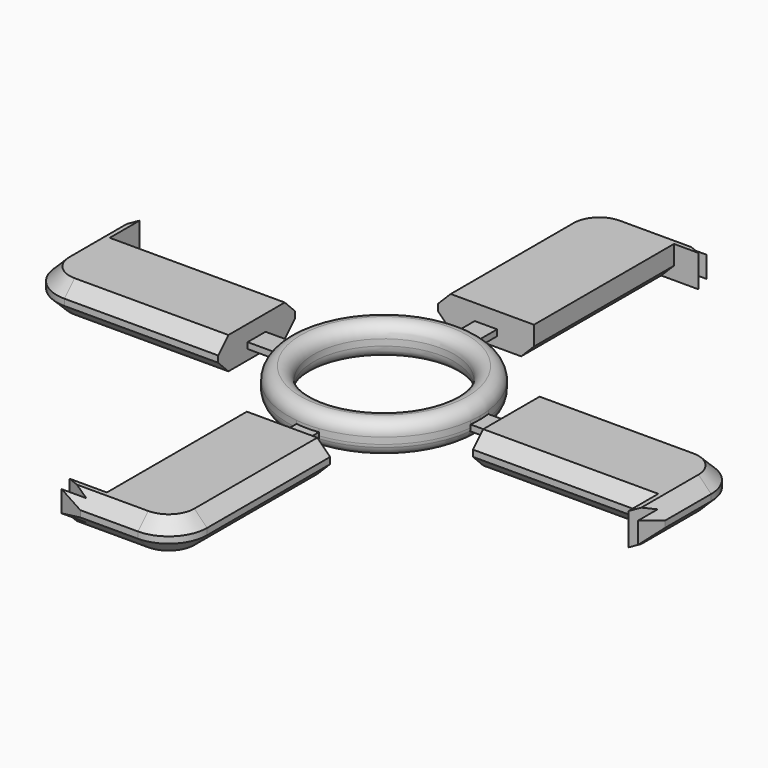
from build123d import *
from build123d import SkipClean  # not in build123d's __all__

# Parameters (mm, degrees)
F1_DEPTH     = 12.7
F0_R         = 27.94
F2_DEPTH     = 6.35
F3_DEPTH     = 3.937
F4_R         = 15.24
F5_SIZE      = 5.08
F6_T9_ANGLE  = 13.3995303555
F6_T16_ANGLE = 76.6004696445
F6_T21_ANGLE = 76.6004696445
F6_T25_ANGLE = 76.6004696445
F6_T30_ANGLE = 76.6004696445
F6_T34_ANGLE = 76.6004696445
F6_T39_ANGLE = 76.6004696445
F6_T43_ANGLE = 76.6004696445
F6_T48_ANGLE = 76.6004696445
F6_T52_ANGLE = 13.3995303555
F6_T56_ANGLE = 13.3995303555
F6_T60_ANGLE = 13.3995303555


# Not quite as in the source:
# - a fillet or chamfer that OpenCascade refuses, or shapes differently, is made with other operations: its cross-section is extruded or revolved along the edge and cut away or added


with BuildPart() as f1:
    # F0 (on Top) → F1 (new body)
    with BuildSketch(Plane.XY):
        Polygon((-50.5398199652, -4.445), (-50.5398199652, 4.445), (-50.5398199652, 19.05), (-119.9662685394, 19.05), (-123.7786710262, 19.05), (-126.7398199652, 19.05), (-126.7398199652, -19.05), (-50.5398199652, -19.05), align=None)
        Polygon((-126.7398199652, 19.05), (-123.7786710262, 19.05), (-123.7786710262, 28.8333185017), align=None)
        Polygon((-123.7786710262, 19.05), (-119.9662685394, 19.05), (-119.9662685394, 28.8333185017), align=None)
    extrude(amount=F1_DEPTH)



with BuildPart() as f1b:
    # F0 (on Top) → F1, piece 2 (new body)
    with BuildSketch(Plane.XY):
        with BuildLine():
            ThreePointArc((37.8398199652, -4.445), (38.0348993733, -2.2263040364), (38.1, 0))
            ThreePointArc((38.1, 0), (38.0348993733, 2.2263040364), (37.8398199652, 4.445))
            ThreePointArc((37.8398199652, 4.445), (26.9407683632, 26.9407683632), (4.445, 37.8398199652))
            ThreePointArc((4.445, 37.8398199652), (0, 38.1), (-4.445, 37.8398199652))
            ThreePointArc((-4.445, 37.8398199652), (-26.9407683632, 26.9407683632), (-37.8398199652, 4.445))
            ThreePointArc((-37.8398199652, 4.445), (-38.1, 0), (-37.8398199652, -4.445))
            ThreePointArc((-37.8398199652, -4.445), (-26.9407683632, -26.9407683632), (-4.445, -37.8398199652))
            ThreePointArc((-4.445, -37.8398199652), (0, -38.1), (4.445, -37.8398199652))
            ThreePointArc((4.445, -37.8398199652), (26.9407683632, -26.9407683632), (37.8398199652, -4.445))
        make_face()
        Circle(F0_R, mode=Mode.SUBTRACT)
    extrude(amount=F1_DEPTH)


with BuildPart() as f1c:
    # F0 (on Top) → F1, piece 3 (new body)
    with BuildSketch(Plane.XY):
        Polygon((50.5398199652, 19.05), (50.5398199652, 4.445), (50.5398199652, -4.445), (50.5398199652, -19.05), (119.9662685394, -19.05), (123.7786710262, -19.05), (126.7398199652, -19.05), (126.7398199652, 19.05), align=None)
        Polygon((123.7786710262, -19.05), (119.9662685394, -19.05), (119.9662685394, -28.8333185017), align=None)
        Polygon((123.7786710262, -28.8333185017), (126.7398199652, -19.05), (123.7786710262, -19.05), align=None)
    extrude(amount=F1_DEPTH)


with BuildPart() as f1d:
    # F0 (on Top) → F1, piece 4 (new body)
    with BuildSketch(Plane.XY):
        Polygon((-4.445, 50.5398199652), (4.445, 50.5398199652), (19.05, 50.5398199652), (19.05, 119.9662685394), (19.05, 123.7786710262), (19.05, 126.7398199652), (-19.05, 126.7398199652), (-19.05, 50.5398199652), align=None)
        Polygon((19.05, 126.7398199652), (19.05, 123.7786710262), (28.8333185017, 123.7786710262), align=None)
        Polygon((19.05, 123.7786710262), (19.05, 119.9662685394), (28.8333185017, 119.9662685394), align=None)
    extrude(amount=F1_DEPTH)


with BuildPart() as f1e:
    # F0 (on Top) → F1, piece 5 (new body)
    with BuildSketch(Plane.XY):
        Polygon((19.05, -50.5398199652), (4.445, -50.5398199652), (-4.445, -50.5398199652), (-19.05, -50.5398199652), (-19.05, -119.9662685394), (-19.05, -123.7786710262), (-19.05, -126.7398199652), (19.05, -126.7398199652), align=None)
        Polygon((-28.8333185017, -123.7786710262), (-19.05, -126.7398199652), (-19.05, -123.7786710262), align=None)
        Polygon((-19.05, -123.7786710262), (-19.05, -119.9662685394), (-28.8333185017, -119.9662685394), align=None)
    extrude(amount=F1_DEPTH)


with BuildPart() as f1_1:
    add(f1.part, clean=False)

    add(f1b.part)  # F2 merges F1b

    add(f1c.part)  # F2 merges F1c

    add(f1d.part)  # F2 merges F1d

    add(f1e.part)  # F2 merges F1e
    # F0 (on Top) → F2 (join)
    with BuildSketch(Plane.XY):
        with BuildLine():
            ThreePointArc((-37.8398199652, -4.445), (-38.1, 0), (-37.8398199652, 4.445))
            Line((-37.8398199652, 4.445), (-50.5398199652, 4.445))
            Line((-50.5398199652, 4.445), (-50.5398199652, -4.445))
            Line((-50.5398199652, -4.445), (-37.8398199652, -4.445))
        make_face()
        with BuildLine():
            ThreePointArc((-4.445, 37.8398199652), (0, 38.1), (4.445, 37.8398199652))
            Line((4.445, 37.8398199652), (4.445, 50.5398199652))
            Line((4.445, 50.5398199652), (-4.445, 50.5398199652))
            Line((-4.445, 50.5398199652), (-4.445, 37.8398199652))
        make_face()
        with BuildLine():
            ThreePointArc((37.8398199652, 4.445), (38.0348993733, 2.2263040364), (38.1, 0))
            ThreePointArc((38.1, 0), (38.0348993733, -2.2263040364), (37.8398199652, -4.445))
            Line((37.8398199652, -4.445), (50.5398199652, -4.445))
            Line((50.5398199652, -4.445), (50.5398199652, 4.445))
            Line((50.5398199652, 4.445), (37.8398199652, 4.445))
        make_face()
        with BuildLine():
            Line((4.445, -50.5398199652), (4.445, -37.8398199652))
            ThreePointArc((4.445, -37.8398199652), (0, -38.1), (-4.445, -37.8398199652))
            Line((-4.445, -37.8398199652), (-4.445, -50.5398199652))
            Line((-4.445, -50.5398199652), (4.445, -50.5398199652))
        make_face()
    extrude(amount=F2_DEPTH)

    # F0 (on Top) → F3 (cut)
    with BuildSketch(Plane.XY):
        with BuildLine():
            Line((4.445, -50.5398199652), (4.445, -37.8398199652))
            ThreePointArc((4.445, -37.8398199652), (0, -38.1), (-4.445, -37.8398199652))
            Line((-4.445, -37.8398199652), (-4.445, -50.5398199652))
            Line((-4.445, -50.5398199652), (4.445, -50.5398199652))
        make_face()
        with BuildLine():
            ThreePointArc((37.8398199652, 4.445), (38.0348993733, 2.2263040364), (38.1, 0))
            ThreePointArc((38.1, 0), (38.0348993733, -2.2263040364), (37.8398199652, -4.445))
            Line((37.8398199652, -4.445), (50.5398199652, -4.445))
            Line((50.5398199652, -4.445), (50.5398199652, 4.445))
            Line((50.5398199652, 4.445), (37.8398199652, 4.445))
        make_face()
        with BuildLine():
            ThreePointArc((-4.445, 37.8398199652), (0, 38.1), (4.445, 37.8398199652))
            Line((4.445, 37.8398199652), (4.445, 50.5398199652))
            Line((4.445, 50.5398199652), (-4.445, 50.5398199652))
            Line((-4.445, 50.5398199652), (-4.445, 37.8398199652))
        make_face()
        with BuildLine():
            ThreePointArc((-37.8398199652, -4.445), (-38.1, 0), (-37.8398199652, 4.445))
            Line((-37.8398199652, 4.445), (-50.5398199652, 4.445))
            Line((-50.5398199652, 4.445), (-50.5398199652, -4.445))
            Line((-50.5398199652, -4.445), (-37.8398199652, -4.445))
        make_face()
    with SkipClean():  # cleaning this boolean's faces spoils the solid; the shape is the same uncleaned
        extrude(amount=F3_DEPTH, mode=Mode.SUBTRACT)

    # F4
    f4_edges = [f1_1.edges().sort_by_distance(p)[0] for p in [
        (126.73982, 19.05, 6.35),
        (19.05, -126.73982, 6.35),
        (-19.05, 126.73982, 6.35),
        (-126.73982, -19.05, 6.35),
    ]]
    fillet(f4_edges, radius=F4_R)

    # F5
    f5_edges = [f1_1.edges().sort_by_distance(p)[0] for p in [
        (81.01982, 19.05, 12.7),
        (81.01982, 19.05, 0),
        (7.62, 126.73982, 12.7),
        (-19.05, 81.01982, 0),
        (19.05, 85.253044, 0),
        (85.253044, -19.05, 0),
        (85.253044, -19.05, 12.7),
        (-85.253044, 19.05, 0),
        (-81.01982, -19.05, 0),
        (-81.01982, -19.05, 12.7),
        (-19.05, -85.253044, 0),
        (19.05, -81.01982, 0),
        (19.05, -81.01982, 12.7),
        (-19.05, -85.253044, 12.7),
        (-85.253044, 19.05, 12.7),
        (14.586307, -122.276127, 0),
        (-7.62, -126.73982, 0),
        (14.586307, -122.276127, 12.7),
        (-7.62, -126.73982, 12.7),
        (-122.276127, -14.586307, 0),
        (-126.73982, 7.62, 0),
        (-126.73982, 7.62, 12.7),
        (-122.276127, -14.586307, 12.7),
        (122.276127, 14.586307, 0),
        (126.73982, -7.62, 0),
        (126.73982, -7.62, 12.7),
        (122.276127, 14.586307, 12.7),
        (-14.586307, 122.276127, 0),
        (7.62, 126.73982, 0),
        (-14.586307, 122.276127, 12.7),
        (-19.05, 81.01982, 12.7),
    ]]
    chamfer(f5_edges, length=F5_SIZE)

    # F6: fillet of radius 5.08 on 8 edges, made by hand


with BuildPart() as f6_tool1:
    # F6_s2 → F6_t3 (revolve)
    with BuildSketch(Plane.XZ):
        with BuildLine():
            ThreePointArc((33.02, 12.7), (29.4278975516, 11.2121024484), (27.94, 7.62))
            Line((27.94, 7.62), (27.94, 12.7))
            Line((27.94, 12.7), (33.02, 12.7))
        make_face()
    revolve(axis=Axis((0, 0, 12.7), (0, 0, 1)))


with BuildPart() as f6_tool4:
    # F6_s5 → F6_t6 (revolve)
    with BuildSketch(Plane(origin=(0, 0, 0), x_dir=(0, 0, 1), z_dir=(-0.1166666667, -0.9931711277, 0))):
        with BuildLine():
            ThreePointArc((7.62, 38.1), (11.2121024484, 36.6121024484), (12.7, 33.02))
            Line((12.7, 33.02), (12.7, 38.1))
            Line((12.7, 38.1), (7.62, 38.1))
        make_face()
    revolve(axis=Axis((0, 0, 12.7), (0, 0, -1)))


with BuildPart() as f6_tool7:
    # F6_s8 → F6_t9 (revolve)
    with BuildSketch(Plane(origin=(0, 0, 0), x_dir=(0, 0, 1), z_dir=(0.1166666667, -0.9931711277, 0))):
        with BuildLine():
            ThreePointArc((5.08, 38.1), (1.4878975516, 36.6121024484), (0, 33.02))
            Line((0, 33.02), (0, 38.1))
            Line((0, 38.1), (5.08, 38.1))
        make_face()
    revolve(axis=Axis((0, 0, 0), (0, 0, -1)), revolution_arc=F6_T9_ANGLE)

    split(bisect_by=Plane.XY.offset(3.937), keep=Keep.BOTTOM)


with BuildPart() as f6_tool11:
    # F6_s12 → F6_t13 (revolve)
    with BuildSketch(Plane.XZ):
        with BuildLine():
            ThreePointArc((33.02, 0), (29.4278975516, 1.4878975516), (27.94, 5.08))
            Line((27.94, 5.08), (27.94, 0))
            Line((27.94, 0), (33.02, 0))
        make_face()
    revolve(axis=Axis((0, 0, 0), (0, 0, 1)))


with BuildPart() as f6_tool14:
    # F6_s15 → F6_t16 (revolve)
    with BuildSketch(Plane(origin=(0, 0, 0), x_dir=(0, 0, 1), z_dir=(-0.1166666667, 0.9931711277, 0))):
        with BuildLine():
            ThreePointArc((5.08, -38.1), (1.4878975516, -36.6121024484), (0, -33.02))
            Line((0, -33.02), (0, -38.1))
            Line((0, -38.1), (5.08, -38.1))
        make_face()
    revolve(axis=Axis((0, 0, 0), (0, 0, 1)), revolution_arc=F6_T16_ANGLE)

    split(bisect_by=Plane.YZ.offset(-4.445), keep=Keep.BOTTOM)

    split(bisect_by=Plane.XZ.offset(4.445), keep=Keep.TOP)


with BuildPart() as f6_tool19:
    # F6_s20 → F6_t21 (revolve)
    with BuildSketch(Plane(origin=(0, 0, 0), x_dir=(0, 0, 1), z_dir=(-0.1166666667, 0.9931711277, 0))):
        with BuildLine():
            ThreePointArc((5.08, -38.1), (1.4878975516, -36.6121024484), (0, -33.02))
            Line((0, -33.02), (0, -38.1))
            Line((0, -38.1), (5.08, -38.1))
        make_face()
    revolve(axis=Axis((0, 0, 0), (0, 0, 1)), revolution_arc=F6_T21_ANGLE)

    split(bisect_by=Plane.XY.offset(3.937), keep=Keep.BOTTOM)


with BuildPart() as f6_tool23:
    # F6_s24 → F6_t25 (revolve)
    with BuildSketch(Plane(origin=(0, 0, 0), x_dir=(0, 0, 1), z_dir=(-0.9931711277, -0.1166666667, 0))):
        with BuildLine():
            ThreePointArc((5.08, -38.1), (1.4878975516, -36.6121024484), (0, -33.02))
            Line((0, -33.02), (0, -38.1))
            Line((0, -38.1), (5.08, -38.1))
        make_face()
    revolve(axis=Axis((0, 0, 0), (0, 0, 1)), revolution_arc=F6_T25_ANGLE)

    split(bisect_by=Plane.YZ.offset(4.445), keep=Keep.TOP)

    split(bisect_by=Plane.XZ.offset(4.445), keep=Keep.TOP)


with BuildPart() as f6_tool28:
    # F6_s29 → F6_t30 (revolve)
    with BuildSketch(Plane(origin=(0, 0, 0), x_dir=(0, 0, 1), z_dir=(-0.9931711277, -0.1166666667, 0))):
        with BuildLine():
            ThreePointArc((5.08, -38.1), (1.4878975516, -36.6121024484), (0, -33.02))
            Line((0, -33.02), (0, -38.1))
            Line((0, -38.1), (5.08, -38.1))
        make_face()
    revolve(axis=Axis((0, 0, 0), (0, 0, 1)), revolution_arc=F6_T30_ANGLE)

    split(bisect_by=Plane.XY.offset(3.937), keep=Keep.BOTTOM)


with BuildPart() as f6_tool32:
    # F6_s33 → F6_t34 (revolve)
    with BuildSketch(Plane(origin=(0, 0, 0), x_dir=(0, 0, 1), z_dir=(0.1166666667, -0.9931711277, 0))):
        with BuildLine():
            ThreePointArc((5.08, -38.1), (1.4878975516, -36.6121024484), (0, -33.02))
            Line((0, -33.02), (0, -38.1))
            Line((0, -38.1), (5.08, -38.1))
        make_face()
    revolve(axis=Axis((0, 0, 0), (0, 0, 1)), revolution_arc=F6_T34_ANGLE)

    split(bisect_by=Plane.XZ.offset(-4.445), keep=Keep.BOTTOM)

    split(bisect_by=Plane.YZ.offset(4.445), keep=Keep.TOP)


with BuildPart() as f6_tool37:
    # F6_s38 → F6_t39 (revolve)
    with BuildSketch(Plane(origin=(0, 0, 0), x_dir=(0, 0, 1), z_dir=(0.1166666667, -0.9931711277, 0))):
        with BuildLine():
            ThreePointArc((5.08, -38.1), (1.4878975516, -36.6121024484), (0, -33.02))
            Line((0, -33.02), (0, -38.1))
            Line((0, -38.1), (5.08, -38.1))
        make_face()
    revolve(axis=Axis((0, 0, 0), (0, 0, 1)), revolution_arc=F6_T39_ANGLE)

    split(bisect_by=Plane.XY.offset(3.937), keep=Keep.BOTTOM)


with BuildPart() as f6_tool41:
    # F6_s42 → F6_t43 (revolve)
    with BuildSketch(Plane(origin=(0, 0, 0), x_dir=(0, 0, 1), z_dir=(0.9931711277, 0.1166666667, 0))):
        with BuildLine():
            ThreePointArc((5.08, -38.1), (1.4878975516, -36.6121024484), (0, -33.02))
            Line((0, -33.02), (0, -38.1))
            Line((0, -38.1), (5.08, -38.1))
        make_face()
    revolve(axis=Axis((0, 0, 0), (0, 0, 1)), revolution_arc=F6_T43_ANGLE)

    split(bisect_by=Plane.YZ.offset(-4.445), keep=Keep.BOTTOM)

    split(bisect_by=Plane.XZ.offset(-4.445), keep=Keep.BOTTOM)


with BuildPart() as f6_tool46:
    # F6_s47 → F6_t48 (revolve)
    with BuildSketch(Plane(origin=(0, 0, 0), x_dir=(0, 0, 1), z_dir=(0.9931711277, 0.1166666667, 0))):
        with BuildLine():
            ThreePointArc((5.08, -38.1), (1.4878975516, -36.6121024484), (0, -33.02))
            Line((0, -33.02), (0, -38.1))
            Line((0, -38.1), (5.08, -38.1))
        make_face()
    revolve(axis=Axis((0, 0, 0), (0, 0, 1)), revolution_arc=F6_T48_ANGLE)

    split(bisect_by=Plane.XY.offset(3.937), keep=Keep.BOTTOM)


with BuildPart() as f6_tool50:
    # F6_s51 → F6_t52 (revolve)
    with BuildSketch(Plane(origin=(0, 0, 0), x_dir=(0, 0, 1), z_dir=(-0.9931711277, -0.1166666667, 0))):
        with BuildLine():
            ThreePointArc((0, 33.02), (1.4878975516, 36.6121024484), (5.08, 38.1))
            Line((5.08, 38.1), (0, 38.1))
            Line((0, 38.1), (0, 33.02))
        make_face()
    revolve(axis=Axis((0, 0, 0), (0, 0, -1)), revolution_arc=F6_T52_ANGLE)

    split(bisect_by=Plane.XY.offset(3.937), keep=Keep.BOTTOM)


with BuildPart() as f6_tool54:
    # F6_s55 → F6_t56 (revolve)
    with BuildSketch(Plane(origin=(0, 0, 0), x_dir=(0, 0, 1), z_dir=(-0.1166666667, 0.9931711277, 0))):
        with BuildLine():
            ThreePointArc((0, 33.02), (1.4878975516, 36.6121024484), (5.08, 38.1))
            Line((5.08, 38.1), (0, 38.1))
            Line((0, 38.1), (0, 33.02))
        make_face()
    revolve(axis=Axis((0, 0, 0), (0, 0, -1)), revolution_arc=F6_T56_ANGLE)

    split(bisect_by=Plane.XY.offset(3.937), keep=Keep.BOTTOM)


with BuildPart() as f6_tool58:
    # F6_s59 → F6_t60 (revolve)
    with BuildSketch(Plane(origin=(0, 0, 0), x_dir=(0, 0, 1), z_dir=(0.9931711277, 0.1166666667, 0))):
        with BuildLine():
            ThreePointArc((5.08, 38.1), (1.4878975516, 36.6121024484), (0, 33.02))
            Line((0, 33.02), (0, 38.1))
            Line((0, 38.1), (5.08, 38.1))
        make_face()
    revolve(axis=Axis((0, 0, 0), (0, 0, -1)), revolution_arc=F6_T60_ANGLE)

    split(bisect_by=Plane.XY.offset(3.937), keep=Keep.BOTTOM)


with BuildPart() as f1_2:
    add(f1_1.part, clean=False)

    # F6_t62: cut F6_tool1, F6_tool4, F6_tool7, F6_tool11, F6_tool14, F6_tool19, F6_tool23, F6_tool28, F6_tool32, F6_tool37, F6_tool41, F6_tool46, F6_tool50, F6_tool54, F6_tool58
    add([f6_tool1.part, f6_tool4.part, f6_tool7.part, f6_tool11.part, f6_tool14.part, f6_tool19.part, f6_tool23.part, f6_tool28.part, f6_tool32.part, f6_tool37.part, f6_tool41.part, f6_tool46.part, f6_tool50.part, f6_tool54.part, f6_tool58.part], mode=Mode.SUBTRACT)


solid = f1_2.part
